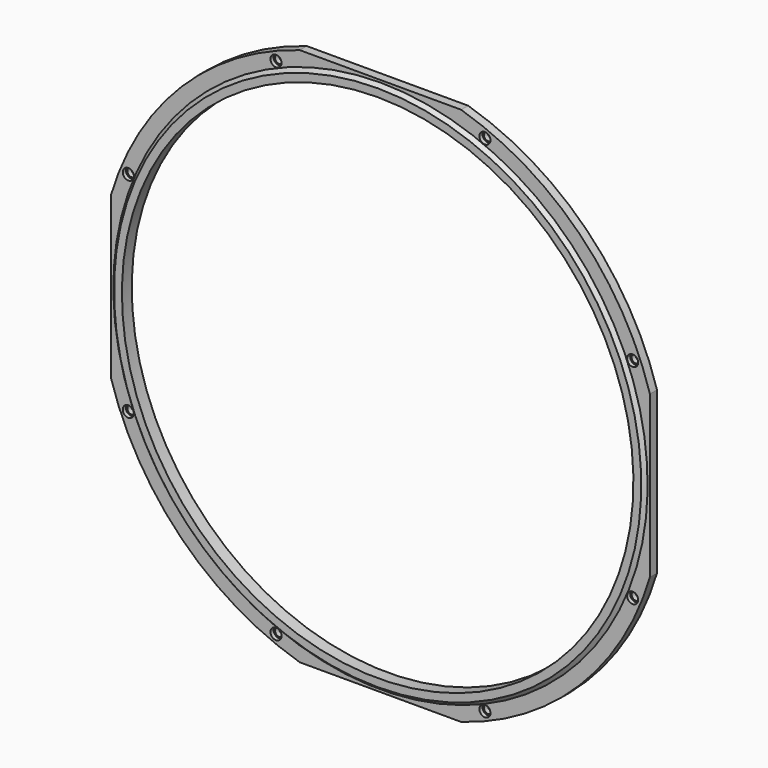
from build123d import *

# Parameters (mm, degrees)
F3_D            = 5.9944
F3_DEPTH        = 25.4
F3_CBORE_D      = 8.001
F3_CBORE_DEPTH  = 2.8448
F3_TIP          = 1.8008994473
F3_COPIES_COUNT = 8
F4_R            = 365.4109378698
F4_W            = 388
F4_H            = 388
F5_DEPTH        = 6.351


# Not quite as in the source:
# - a pattern or mirror of a feature is missing from the dataset's text; its kind, count and spacing are read off the source's solid


with BuildPart() as f1:
    # F0 (on Right) → F1 (revolve)
    with BuildSketch(Plane.YZ):
        Polygon((-8.89, 184.15), (0, 184.15), (0, 202.5), (-6.35, 202.5), (-6.35, 192.34), (-8.89, 189.8), align=None)
    revolve(axis=Axis((0, 77.3353951023, 0), (0, 1, 0)))

    # F3
    with Locations(Plane.XZ.offset(6.35)):
        with Locations((75.1972944597, 181.5423281385)):
            f3 = CounterBoreHole(F3_D / 2, F3_CBORE_D / 2, F3_CBORE_DEPTH, depth=F3_DEPTH)
            with Locations((0, 0, -(F3_DEPTH + F3_TIP / 2))):  # 118° drill point
                Cone(0, F3_D / 2, F3_TIP, mode=Mode.SUBTRACT)

    # F3_copies: F3 ×8 about axis
    f3_copies_axis = Axis((0, 0, 0), (0, 1, 0))
    for i in range(1, F3_COPIES_COUNT):
        add(f3.rotate(f3_copies_axis, i * 360 / F3_COPIES_COUNT), mode=Mode.SUBTRACT)

    # F4 (on face) → F5 (cut, through all)
    with BuildSketch(Plane.XZ.offset(6.35)):
        Circle(F4_R)
        Rectangle(F4_W, F4_H, mode=Mode.SUBTRACT)
    extrude(amount=-F5_DEPTH, mode=Mode.SUBTRACT)


solid = f1.part
